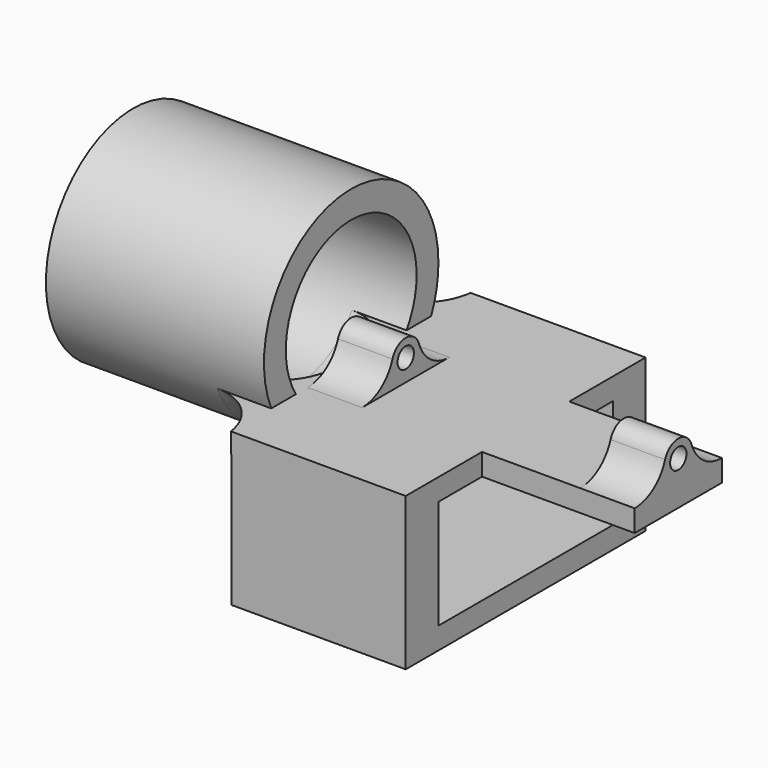
from build123d import *

# Parameters (mm, degrees)
F0_R        = 12.7
F0_R_2      = 9.525
F1_DEPTH    = 25.4
F2_W        = 34.925
F2_H        = 17.78
F2_W_2      = 25.4
F2_H_2      = 12.7
F3_DEPTH    = 2.54
F4_DEPTH    = 20.32
F5_T4_ANGLE = 306.6504874214
F5_T9_ANGLE = 276.2084965167
F6_W        = 12.7
F6_H        = 2.54
F7_DEPTH    = 17.78
F8_R        = 1.190625
F9_DEPTH    = 38.1
F10_W       = 25.4
F10_H       = 5.08
F11_DEPTH   = 12.7


# Not quite as in the source:
# - a fillet or chamfer that OpenCascade refuses, or shapes differently, is made with other operations: its cross-section is extruded or revolved along the edge and cut away or added


with BuildPart() as f1:
    # F0 (on Right) → F1 (new body)
    with BuildSketch(Plane.YZ):
        Circle(F0_R)
        Circle(F0_R_2, mode=Mode.SUBTRACT)
    extrude(amount=-F1_DEPTH)

    # F2 (on Right) → F3 (join)
    with BuildSketch(Plane.YZ):
        with Locations((0, -13.97)):
            Rectangle(F2_W, F2_H)
        with Locations((0, -13.97)):
            Rectangle(F2_W_2, F2_H_2, mode=Mode.SUBTRACT)
        with Locations((0, -13.97)):
            Rectangle(F2_W_2, F2_H_2)
    extrude(amount=F3_DEPTH)

    # F2 (on Right) → F4 (join)
    with BuildSketch(Plane.YZ):
        with Locations((0, -13.97)):
            Rectangle(F2_W, F2_H)
        with Locations((0, -13.97)):
            Rectangle(F2_W_2, F2_H_2, mode=Mode.SUBTRACT)
    extrude(amount=F4_DEPTH)

    # F5: fillet of radius 6.35 on 2 edges, made by hand


with BuildPart() as f5_tool2:
    # F5_s3 → F5_t4 (revolve)
    with BuildSketch(Plane(origin=(0, 0, 0), x_dir=(1, 0, 0), z_dir=(0, 0.8935692652, 0.4489253482))):
        with BuildLine():
            ThreePointArc((-6.35, -9.525), (-1.8598719395, -7.6651280605), (0, -3.175))
            Line((0, -3.175), (0, -9.525))
            Line((0, -9.525), (-6.35, -9.525))
        make_face()
    revolve(axis=Axis((0, 0, 0), (1, 0, 0)), revolution_arc=F5_T4_ANGLE)

    split(bisect_by=Plane.XY.offset(-5.08), keep=Keep.BOTTOM)


with BuildPart() as f1_1:
    add(f1.part)

    # F5_t1: union F5_tool2
    add(f5_tool2.part)


with BuildPart() as f5_tool7:
    # F5_s8 → F5_t9 (revolve)
    with BuildSketch(Plane(origin=(0, 0, 0), x_dir=(1, 0, 0), z_dir=(0, -0.7443610614, 0.6677773658))):
        with BuildLine():
            ThreePointArc((-6.35, 12.7), (-1.8598719395, 14.5598719395), (0, 19.05))
            Line((0, 19.05), (0, 12.7))
            Line((0, 12.7), (-6.35, 12.7))
        make_face()
    revolve(axis=Axis((0, 0, 0), (-1, 0, 0)), revolution_arc=F5_T9_ANGLE)

    split(bisect_by=Plane.XY.offset(-5.08), keep=Keep.BOTTOM)

    split(bisect_by=Plane.XZ.offset(17.4625), keep=Keep.BOTTOM)

    split(bisect_by=Plane.XZ.offset(-17.4625), keep=Keep.TOP)


with BuildPart() as f1_2:
    add(f1_1.part)

    # F5_t6: union F5_tool7
    add(f5_tool7.part)

    # F6 (on face) → F7 (join)
    with BuildSketch(Plane.YZ.offset(20.32)):
        with Locations((0, -6.35)):
            Rectangle(F6_W, F6_H)
    extrude(amount=F7_DEPTH)

    # F8 (on face) → F9 (join)
    with BuildSketch(Plane.YZ.offset(38.1)):
        with BuildLine():
            ThreePointArc((1.927081138, -1.8954984194), (0, -0.508), (-1.927081138, -1.8954984194))
            ThreePointArc((-1.927081138, -1.8954984194), (-3.6249650655, -4.2010485201), (-6.35, -5.08))
            Line((-6.35, -5.08), (6.35, -5.08))
            ThreePointArc((6.35, -5.08), (3.6249650655, -4.2010485201), (1.927081138, -1.8954984194))
        make_face()
        with Locations((0, -2.54)):
            Circle(F8_R, mode=Mode.SUBTRACT)
    extrude(amount=-F9_DEPTH)

    # F10 (on Front) → F11 (cut, symmetric)
    with BuildSketch(Plane.XZ):
        with Locations((19.05, -2.54)):
            Rectangle(F10_W, F10_H)
    extrude(amount=F11_DEPTH, both=True, mode=Mode.SUBTRACT)


solid = f1_2.part
